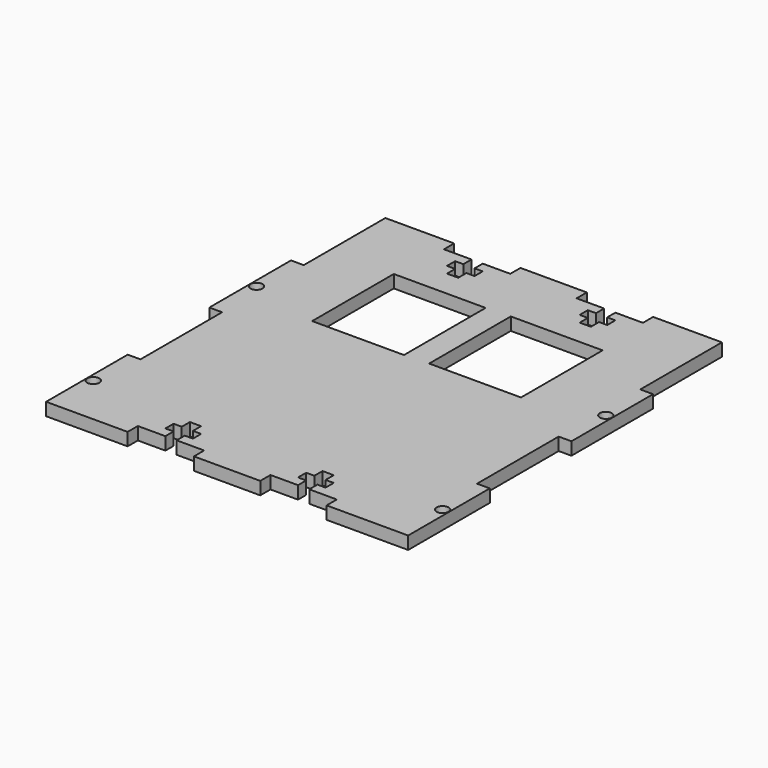
from build123d import *

# Parameters (mm, degrees)
F0_R     = 1.5
F0_W     = 22.86
F0_H     = 25.4
F1_DEPTH = 3.175


# Not quite as in the source:
# - a length typed as a fraction of an inch, garbled in the dataset ("3 / 203.2 mm" for 3/8 in), is restored


with BuildPart() as f1:
    # F0 (on Top) → F1 (new body)
    with BuildSketch(Plane.XY):
        Polygon((-41.8889727067, -63.5), (-24.765, -63.5), (-24.765, -60.325), (-17.907, -60.325), (-17.907, -57.785), (-19.939, -57.785), (-19.939, -55.245), (-17.907, -55.245), (-17.907, -52.705), (-15.113, -52.705), (-15.113, -55.245), (-13.081, -55.245), (-13.081, -57.785), (-15.113, -57.785), (-15.113, -60.325), (-8.255, -60.325), (-8.255, -63.5), (8.255, -63.5), (8.255, -60.325), (15.113, -60.325), (15.113, -57.785), (13.081, -57.785), (13.081, -55.245), (15.113, -55.245), (15.113, -52.705), (17.907, -52.705), (17.907, -55.245), (19.939, -55.245), (19.939, -57.785), (17.907, -57.785), (17.907, -60.325), (24.765, -60.325), (24.765, -63.5), (41.8889727067, -63.5), (41.91, -63.5), (45.0639727067, -63.5), (45.0639727067, -38.1), (41.8889727067, -38.1), (41.8889727067, -12.7), (45.0639727067, -12.7), (45.0639727067, 12.7), (41.8889727067, 12.7), (41.8889727067, 38.1), (24.765, 38.1), (24.765, 34.925), (17.907, 34.925), (17.907, 32.385), (19.939, 32.385), (19.939, 29.845), (17.907, 29.845), (17.907, 27.305), (15.113, 27.305), (15.113, 29.845), (13.081, 29.845), (13.081, 32.385), (15.113, 32.385), (15.113, 34.925), (8.255, 34.925), (8.255, 38.1), (-8.255, 38.1), (-8.255, 34.925), (-15.113, 34.925), (-15.113, 32.385), (-13.081, 32.385), (-13.081, 29.845), (-15.113, 29.845), (-15.113, 27.305), (-17.907, 27.305), (-17.907, 29.845), (-19.939, 29.845), (-19.939, 32.385), (-17.907, 32.385), (-17.907, 34.925), (-24.765, 34.925), (-24.765, 38.1), (-41.8889727067, 38.1), (-41.8889727067, 12.7), (-45.0639727067, 12.7), (-45.0639727067, -12.7), (-41.8889727067, -12.7), (-41.8889727067, -38.1), (-45.0639727067, -38.1), (-45.0639727067, -63.5), (-41.91, -63.5), align=None)
        with Locations((-43.4764727067, -50.8)):
            Circle(F0_R, mode=Mode.SUBTRACT)
        with Locations((43.4764727067, -50.8)):
            Circle(F0_R, mode=Mode.SUBTRACT)
        with Locations((-43.4764727067, 0)):
            Circle(F0_R, mode=Mode.SUBTRACT)
        with Locations((-14.4632559413, 8.0235061839)):
            Rectangle(F0_W, F0_H, mode=Mode.SUBTRACT)
        with Locations((14.4632559413, 8.2762846043)):
            Rectangle(F0_W, F0_H, mode=Mode.SUBTRACT)
        with Locations((43.4764727067, 0)):
            Circle(F0_R, mode=Mode.SUBTRACT)
    extrude(amount=F1_DEPTH)


solid = f1.part
